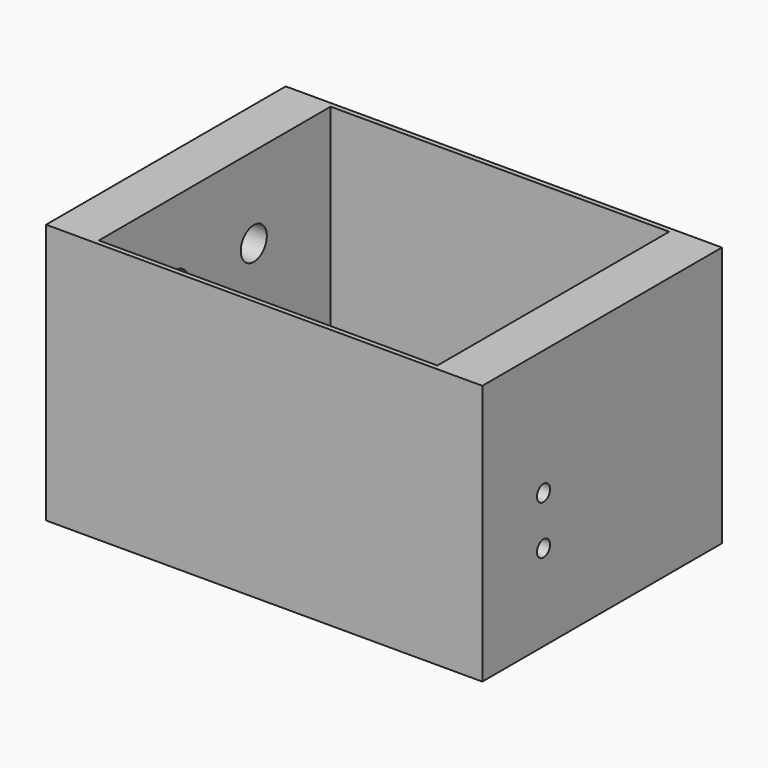
from build123d import *

# Parameters (mm, degrees)
F0_R      = 25.5
F1_DEPTH  = 2
F0_R_2    = 5
F2_DEPTH  = 5
F3_DEPTH  = 160
F4_DEPTH  = 40
F5_R      = 5
F6_DEPTH  = 30.3
F7_DEPTH  = 30
F8_DEPTH  = 10
F9_R      = 10
F10_DEPTH = 30


# Not quite as in the source:
# - a feature names something its author has since deleted; it is built from what else it names


with BuildPart() as f1:
    # F0 (on Top) → F1 (new body)
    with BuildSketch(Plane.XY):
        Circle(F0_R)
    extrude(amount=F1_DEPTH)

    # F0 (on Top) → F8 (cut)
    with BuildSketch(Plane.XY):
        with BuildLine():
            Line((94, 35), (94, 45))
            Line((94, 45), (94, 55))
            ThreePointArc((94, 55), (90, 59), (86, 55))
            Line((86, 55), (86, 35))
            ThreePointArc((86, 35), (90, 31), (94, 35))
        make_face()
    extrude(amount=F8_DEPTH, mode=Mode.SUBTRACT)


with BuildPart() as f2:
    # F0 (on Top) → F2 (new body)
    with BuildSketch(Plane.XY):
        Polygon((100, -40), (100, 45), (100, 130), (-100, 130), (-100, -40), align=None)
        Circle(F0_R, mode=Mode.SUBTRACT)
        with Locations((-94, 45)):
            Circle(F0_R_2, mode=Mode.SUBTRACT)
        with BuildLine():
            Line((94, 55), (94, 45))
            Line((94, 45), (94, 35))
            ThreePointArc((94, 35), (90, 31), (86, 35))
            Line((86, 35), (86, 55))
            ThreePointArc((86, 55), (90, 59), (94, 55))
        make_face(mode=Mode.SUBTRACT)
    extrude(amount=F2_DEPTH)


with BuildPart() as f3:
    # F0 (on Top) → F3 (new body)
    with BuildSketch(Plane.XY):
        Polygon((-134, -47), (134, -47), (134, 45), (134, 137), (-134, 137), align=None)
        Polygon((104, 134), (104, 45), (104, -44), (-104, -44), (-104, 134), align=None, mode=Mode.SUBTRACT)
    extrude(amount=F3_DEPTH)

    # F5 (on face) → F6 (cut)
    with BuildSketch(Plane.YZ.offset(134)):
        with Locations((0, 83)):
            Circle(F5_R)
    extrude(amount=-F6_DEPTH, mode=Mode.SUBTRACT)

    # F5 (on face) → F7 (cut)
    with BuildSketch(Plane.YZ.offset(134)):
        with Locations((0, 53)):
            Circle(F5_R)
    extrude(amount=-F7_DEPTH, mode=Mode.SUBTRACT)

    # F9 (on face) → F10 (cut, through all)
    with BuildSketch(Plane(origin=(-134, 0, 0), x_dir=(0, -1, 0), z_dir=(-1, 0, 0))):
        with Locations((-75, 110)):
            Circle(F9_R)
        with Locations((-15, 110)):
            Circle(F9_R)
        with Locations((-75, 50)):
            Circle(F9_R)
        with Locations((-15, 50)):
            Circle(F9_R)
    extrude(amount=-F10_DEPTH, mode=Mode.SUBTRACT)


with BuildPart() as f4:
    # F0 (on Top) → F4 (new body)
    with BuildSketch(Plane.XY):
        Polygon((104, -44), (104, 45), (104, 134), (-104, 134), (-104, -44), align=None)
        Polygon((100, 130), (100, 45), (100, -40), (-100, -40), (-100, 130), align=None, mode=Mode.SUBTRACT)
    extrude(amount=F4_DEPTH)


solid = Compound([f1.part, f2.part, f3.part, f4.part])
